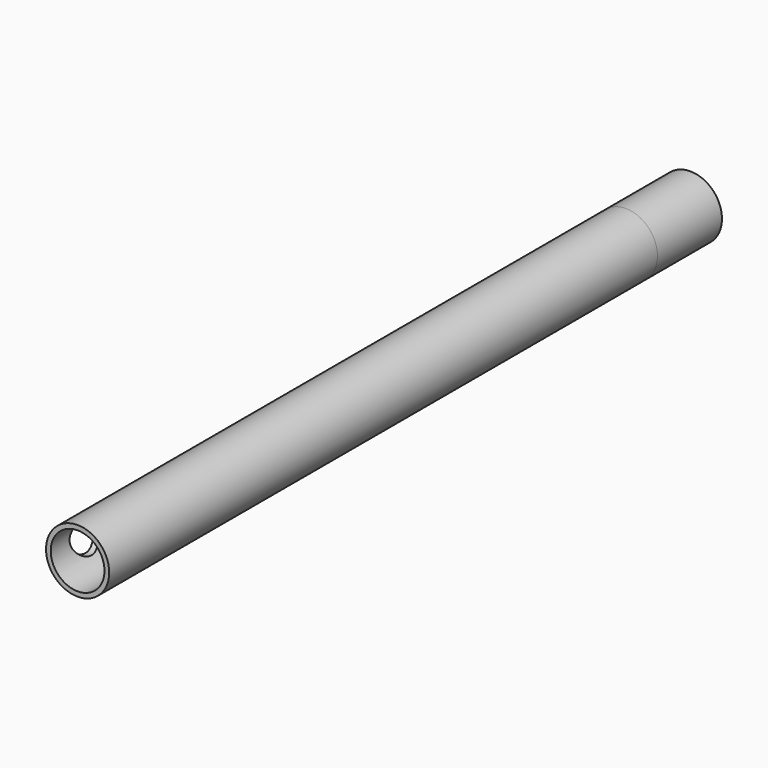
from build123d import *

# Parameters (mm, degrees)
F3_R      = 4.7
F4_DEPTH  = 92
F8_DEPTH  = 92
F6_R      = 4.7
F6_R_2    = 4
F9_DEPTH  = 10
F7_R      = 4.7
F7_R_2    = 4
F10_DEPTH = 12
F11_R     = 2.75
F12_DEPTH = 4.701


# Not quite as in the source:
# - ends of sketch curves that miss each other by under 0.0002 mm in the source are joined


with BuildPart() as f4:
    # F3 (on Front) → F4 (new body)
    with BuildSketch(Plane.XZ):
        Circle(F3_R)
    extrude(amount=F4_DEPTH)

    # F5 (on face) → F8 (cut, through all)
    with BuildSketch(Plane.XZ.offset(92)):
        with BuildLine():
            Line((-1.25, -3.8), (0, -3.8))
            Line((0, -3.8), (1.25, -3.8))
            Line((1.25, -3.8), (1.25, -3.7))
            ThreePointArc((1.25, -3.7), (1.3085786438, -3.5585786438), (1.45, -3.5))
            Line((1.45, -3.5), (2, -3.5))
            Line((2, -3.5), (2, -3.05))
            ThreePointArc((2, -3.05), (2.0585786438, -2.9085786438), (2.2, -2.85))
            Line((2.2, -2.85), (3.15, -2.85))
            Line((3.15, -2.85), (3.15, -2.15))
            Line((3.15, -2.15), (2.2, -2.15))
            ThreePointArc((2.2, -2.15), (2.0585786438, -2.0914213562), (2, -1.95))
            Line((2, -1.95), (2, -1.887459))
            ThreePointArc((2, -1.887459), (2.1033535752, -1.771554046), (2.2, -1.65))
            Line((2.2, -1.65), (3.75, -1.65))
            Line((3.75, -1.65), (3.75, 0))
            Line((3.75, 0), (3.75, 1.65))
            Line((3.75, 1.65), (2.2, 1.65))
            ThreePointArc((2.2, 1.65), (2.1033535752, 1.771554046), (1.9999998047, 1.8874588157))
            Line((1.9999998047, 1.8874588157), (2, 1.95))
            ThreePointArc((2, 1.95), (2.0585786438, 2.0914213562), (2.2, 2.15))
            Line((2.2, 2.15), (3.15, 2.15))
            Line((3.15, 2.15), (3.15, 2.85))
            Line((3.15, 2.85), (2.2, 2.85))
            ThreePointArc((2.2, 2.85), (2.0585786438, 2.9085786438), (2, 3.05))
            Line((2, 3.05), (2, 3.5))
            Line((2, 3.5), (1.45, 3.5))
            ThreePointArc((1.45, 3.5), (1.3085786438, 3.5585786438), (1.25, 3.7))
            Line((1.25, 3.7), (1.25, 3.8))
            Line((1.25, 3.8), (0, 3.8))
            Line((0, 3.8), (-1.25, 3.8))
            Line((-1.25, 3.8), (-1.25, 3.7))
            ThreePointArc((-1.25, 3.7), (-1.3085786438, 3.5585786438), (-1.45, 3.5))
            Line((-1.45, 3.5), (-2, 3.5))
            Line((-2, 3.5), (-2, 3.05))
            ThreePointArc((-2, 3.05), (-2.0585786438, 2.9085786438), (-2.2, 2.85))
            Line((-2.2, 2.85), (-3.15, 2.85))
            Line((-3.15, 2.85), (-3.15, 2.15))
            Line((-3.15, 2.15), (-2.2, 2.15))
            ThreePointArc((-2.2, 2.15), (-2.0585786438, 2.0914213562), (-2, 1.95))
            Line((-2, 1.95), (-2, 1.887459))
            ThreePointArc((-2, 1.887459), (-2.1033535752, 1.771554046), (-2.2, 1.65))
            Line((-2.2, 1.65), (-3.75, 1.65))
            Line((-3.75, 1.65), (-3.75, 0))
            Line((-3.75, 0), (-3.75, -1.65))
            Line((-3.75, -1.65), (-2.2, -1.65))
            ThreePointArc((-2.2, -1.65), (-2.1033535752, -1.771554046), (-1.9999998047, -1.8874588157))
            Line((-1.9999998047, -1.8874588157), (-2, -1.95))
            ThreePointArc((-2, -1.95), (-2.0585786438, -2.0914213562), (-2.2, -2.15))
            Line((-2.2, -2.15), (-3.15, -2.15))
            Line((-3.15, -2.15), (-3.15, -2.85))
            Line((-3.15, -2.85), (-2.2, -2.85))
            ThreePointArc((-2.2, -2.85), (-2.0585786438, -2.9085786438), (-2, -3.05))
            Line((-2, -3.05), (-2, -3.5))
            Line((-2, -3.5), (-1.45, -3.5))
            ThreePointArc((-1.45, -3.5), (-1.3085786438, -3.5585786438), (-1.25, -3.7))
            Line((-1.25, -3.7), (-1.25, -3.8))
        make_face()
    extrude(amount=-F8_DEPTH, mode=Mode.SUBTRACT)

    # F6 (on face) → F9 (join)
    with BuildSketch(Plane.XZ.offset(92)):
        Circle(F6_R)
        Circle(F6_R_2, mode=Mode.SUBTRACT)
    extrude(amount=F9_DEPTH)

    # F7 (on face) → F10 (join)
    with BuildSketch(Plane(origin=(0, 0, 0), x_dir=(-1, 0, 0), z_dir=(0, 1, 0))):
        Circle(F7_R)
        Circle(F7_R_2, mode=Mode.SUBTRACT)
    extrude(amount=F10_DEPTH)

    # F11 (on Right) → F12 (cut, through all)
    with BuildSketch(Plane.YZ):
        with Locations((-95.75, 0)):
            Circle(F11_R)
    extrude(amount=-F12_DEPTH, mode=Mode.SUBTRACT)


solid = f4.part
